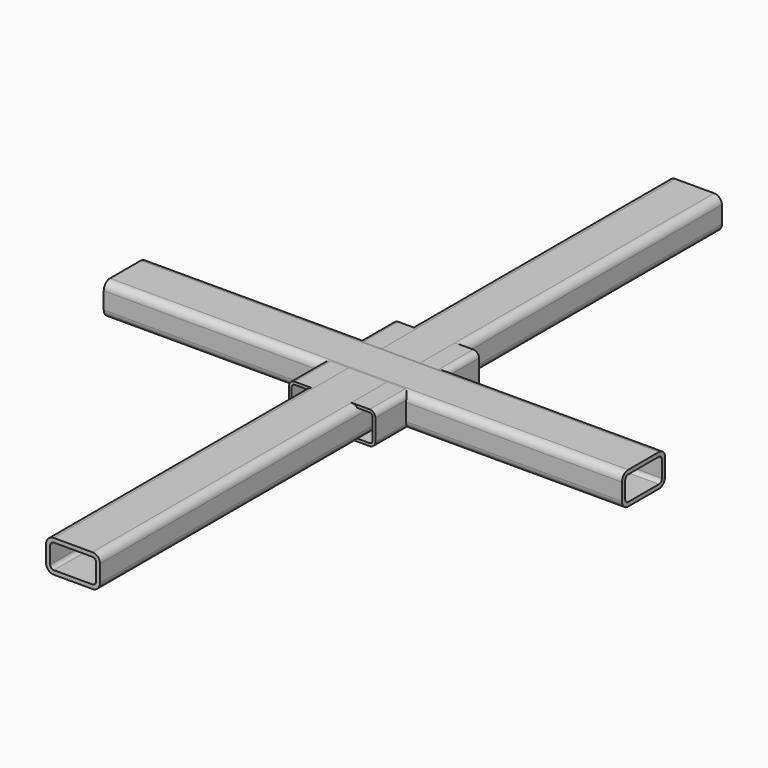
from build123d import *

# Parameters (mm, degrees)
F1_DEPTH  = 152.4
F3_D      = 19.05
F3_DEPTH  = 12.7
F3_TIP    = 5.7231973962
F5_DEPTH  = 16.256
F6_D      = 16.66748
F8_DEPTH  = 914.4
F10_DEPTH = 609.6
F12_DEPTH = 9.525


# Not quite as in the source:
# - ends of sketch curves that miss each other by under 0.0002 mm in the source are joined


with BuildPart() as f1:
    # F0 (on Front) → F1 (new body, symmetric)
    with BuildSketch(Plane.XZ):
        with BuildLine():
            ThreePointArc((101.6, 24.6126), (97.6496320006, 34.1496320006), (88.1126, 38.1))
            Line((88.1126, 38.1), (-88.1126, 38.1))
            ThreePointArc((-88.1126, 38.1), (-97.6496337703, 34.1496337703), (-101.6000025028, 24.6126))
            Line((-101.6000025028, 24.6126), (-101.6, -24.6126))
            ThreePointArc((-101.6, -24.6126), (-97.6496320006, -34.1496320006), (-88.1126, -38.1))
            Line((-88.1126, -38.1), (88.1126, -38.1))
            ThreePointArc((88.1126, -38.1), (97.6496320006, -34.1496320006), (101.6, -24.6126))
            Line((101.6, -24.6126), (101.6, 24.6126))
        make_face()
        with BuildLine():
            ThreePointArc((-95.25, 24.6126), (-93.15950394, 29.65950394), (-88.1126, 31.75))
            Line((-88.1126, 31.75), (88.1126, 31.75))
            ThreePointArc((88.1126, 31.75), (93.15950394, 29.65950394), (95.25, 24.6126))
            Line((95.25, 24.6126), (95.25, -24.6126))
            ThreePointArc((95.25, -24.6126), (93.15950394, -29.65950394), (88.1126, -31.75))
            Line((88.1126, -31.75), (-88.1126, -31.75))
            ThreePointArc((-88.1126, -31.75), (-93.15950394, -29.65950394), (-95.25, -24.6126))
            Line((-95.25, -24.6126), (-95.25, 24.6126))
        make_face(mode=Mode.SUBTRACT)
    extrude(amount=F1_DEPTH, both=True)

    # F3
    with Locations(Plane.YZ.offset(101.6)):
        with Locations((0, 0)):
            Hole(F3_D / 2, depth=F3_DEPTH)
            with Locations((0, 0, -(F3_DEPTH + F3_TIP / 2))):  # 118° drill point
                Cone(0, F3_D / 2, F3_TIP, mode=Mode.SUBTRACT)


with BuildPart() as f5:
    # F4 (on Right) → F5 (new body)
    with BuildSketch(Plane.YZ):
        Polygon((8.0215891701, 13.8938), (-8.0215891701, 13.8938), (-16.0431783401, 0), (-8.0215891701, -13.8938), (8.0215891701, -13.8938), (16.0431783401, 0), align=None)
    extrude(amount=F5_DEPTH)

    # F6 (through all)
    with Locations(Plane(origin=(0, 0, 0), x_dir=(0, 1, 0), z_dir=(-1, 0, 0))):
        with Locations((0, 0)):
            Hole(F6_D / 2)


with BuildPart() as f8:
    # F7 (on Front) → F8 (new body, symmetric)
    with BuildSketch(Plane.XZ):
        with BuildLine():
            Line((45.2628, 38.1), (-45.2628, 38.1))
            ThreePointArc((-45.2628, 38.1), (-58.1584477899, 32.7584477899), (-63.5, 19.8628))
            Line((-63.5, 19.8628), (-63.5, -19.8628))
            ThreePointArc((-63.5, -19.8628), (-58.1584477899, -32.7584477899), (-45.2628, -38.1))
            Line((-45.2628, -38.1), (45.2628, -38.1))
            ThreePointArc((45.2628, -38.1), (58.1584477899, -32.7584477899), (63.5, -19.8628))
            Line((63.5, -19.8628), (63.5, 19.8628))
            ThreePointArc((63.5, 19.8628), (58.1584477899, 32.7584477899), (45.2628, 38.1))
        make_face()
        with BuildLine():
            Line((45.2628, -28.575), (-45.2628, -28.575))
            ThreePointArc((-45.2628, -28.575), (-51.4232556991, -26.0232556991), (-53.975, -19.8628))
            Line((-53.975, -19.8628), (-53.975, 19.8628))
            ThreePointArc((-53.975, 19.8628), (-51.4232556991, 26.0232556991), (-45.2628, 28.575))
            Line((-45.2628, 28.575), (45.2628, 28.575))
            ThreePointArc((45.2628, 28.575), (51.4232556991, 26.0232556991), (53.975, 19.8628))
            Line((53.975, 19.8628), (53.975, -19.8628))
            ThreePointArc((53.975, -19.8628), (51.4232556991, -26.0232556991), (45.2628, -28.575))
        make_face(mode=Mode.SUBTRACT)
    extrude(amount=F8_DEPTH, both=True)


with BuildPart() as f10:
    # F9 (on Right) → F10 (new body, symmetric)
    with BuildSketch(Plane.YZ):
        with BuildLine():
            Line((46.5726517666, 38.427462476), (-43.9529482334, 38.427462476))
            ThreePointArc((-43.9529482334, 38.427462476), (-56.8485960233, 33.0859102658), (-62.1901482334, 20.190262476))
            Line((-62.1901482334, 20.190262476), (-62.1901482334, -19.535337524))
            ThreePointArc((-62.1901482334, -19.535337524), (-56.8485960233, -32.4309853139), (-43.9529482334, -37.772537524))
            Line((-43.9529482334, -37.772537524), (46.5726517666, -37.772537524))
            ThreePointArc((46.5726517666, -37.772537524), (59.4682995564, -32.4309853139), (64.8098517666, -19.535337524))
            Line((64.8098517666, -19.535337524), (64.8098517666, 20.190262476))
            ThreePointArc((64.8098517666, 20.190262476), (59.4682995564, 33.0859102658), (46.5726517666, 38.427462476))
        make_face()
        with BuildLine():
            Line((46.5726517666, -28.247537524), (-43.9529482334, -28.247537524))
            ThreePointArc((-43.9529482334, -28.247537524), (-50.1134039325, -25.6957932231), (-52.6651482334, -19.535337524))
            Line((-52.6651482334, -19.535337524), (-52.6651482334, 20.190262476))
            ThreePointArc((-52.6651482334, 20.190262476), (-50.1134039325, 26.350718175), (-43.9529482334, 28.902462476))
            Line((-43.9529482334, 28.902462476), (46.5726517666, 28.902462476))
            ThreePointArc((46.5726517666, 28.902462476), (52.7331074656, 26.350718175), (55.2848517666, 20.190262476))
            Line((55.2848517666, 20.190262476), (55.2848517666, -19.535337524))
            ThreePointArc((55.2848517666, -19.535337524), (52.7331074656, -25.6957932231), (46.5726517666, -28.247537524))
        make_face(mode=Mode.SUBTRACT)
    extrude(amount=F10_DEPTH, both=True)


with BuildPart() as f12:
    # F11 (on Front) → F12 (new body)
    with BuildSketch(Plane.XZ):
        with BuildLine():
            ThreePointArc((-54.1933096803, -19.7536458365), (-51.6415653794, -25.9141015355), (-45.4811096803, -28.4658458365))
            Line((-45.4811096803, -28.4658458365), (45.0444903197, -28.4658458365))
            ThreePointArc((45.0444903197, -28.4658458365), (51.2049460187, -25.9141015355), (53.7566903197, -19.7536458365))
            Line((53.7566903197, -19.7536458365), (53.7566903197, 19.9719541635))
            ThreePointArc((53.7566903197, 19.9719541635), (51.2049460187, 26.1324098626), (45.0444903197, 28.6841541635))
            Line((45.0444903197, 28.6841541635), (-45.4811096803, 28.6841541635))
            ThreePointArc((-45.4811096803, 28.6841541635), (-51.6415653794, 26.1324098626), (-54.1933096803, 19.9719541635))
            Line((-54.1933096803, 19.9719541635), (-54.1933096803, -19.7536458365))
        make_face()
    extrude(amount=F12_DEPTH)


solid = Compound([f1.part, f5.part, f8.part, f10.part, f12.part])
